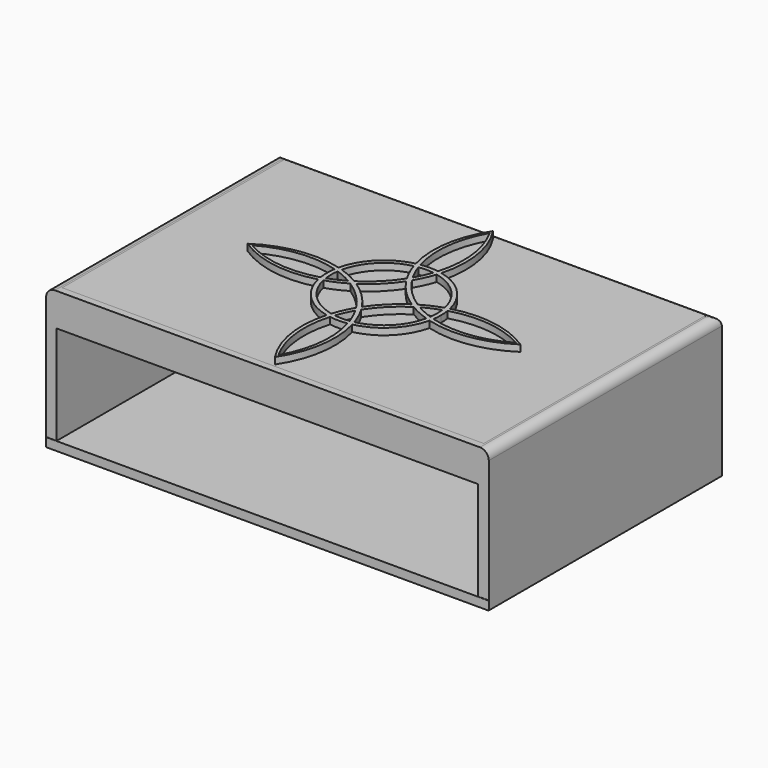
from build123d import *

# Parameters (mm, degrees)
F1_DEPTH    = 3.81
F8_DEPTH    = 81.28
F2_W        = 243.4270217588
F2_H        = 4.0062579512
F5_DEPTH    = 19.05
F2_H_2      = 160.2307879926
F6_DEPTH    = 5.08
F4_W        = 255.387352037
F4_H        = 168.597304807
F9_DEPTH    = 5.08
F7_T1_DEPTH = 193.643303895
F7_T3_DEPTH = 280.9998563766


# Not quite as in the source:
# - a fillet or chamfer that OpenCascade refuses, or shapes differently, is made with other operations: its cross-section is extruded or revolved along the edge and cut away or added


with BuildPart() as f1:
    # F0 (on Top) → F1 (new body)
    with BuildSketch(Plane.XY):
        with BuildLine():
            ThreePointArc((7.3915821042, -32.1820588837), (23.3486659148, -23.3486659148), (32.1820588837, -7.3915821042))
            ThreePointArc((32.1820588837, -7.3915821042), (30.9590231559, -7.0377991533), (29.7442225234, -6.6566978658))
            ThreePointArc((29.7442225234, -6.6566978658), (21.5526146906, -21.5526146906), (6.6566978658, -29.7442225234))
            ThreePointArc((6.6566978658, -29.7442225234), (7.0377991533, -30.9590231559), (7.3915821042, -32.1820588837))
        make_face()
        with BuildLine():
            ThreePointArc((29.7442225234, -6.6566978658), (30.9590231559, -7.0377991533), (32.1820588837, -7.3915821042))
            ThreePointArc((32.1820588837, -7.3915821042), (32.4249296069, -6.2405400398), (32.6266451411, -5.0815771994))
            ThreePointArc((32.6266451411, -5.0815771994), (31.3967387773, -4.7023200855), (30.1759000362, -4.294817459))
            ThreePointArc((30.1759000362, -4.294817459), (29.9833268944, -5.4800098856), (29.7442225234, -6.6566978658))
        make_face()
        with BuildLine():
            ThreePointArc((33.02, 0), (32.9215144135, 2.5483894364), (32.6266451411, 5.0815771994))
            ThreePointArc((32.6266451411, 5.0815771994), (31.3967387773, 4.7023200855), (30.1759000362, 4.294817459))
            ThreePointArc((30.1759000362, 4.294817459), (30.4038799588, 2.1527850447), (30.48, 0))
            ThreePointArc((30.48, 0), (30.4038799588, -2.1527850447), (30.1759000362, -4.294817459))
            ThreePointArc((30.1759000362, -4.294817459), (31.3967387773, -4.7023200855), (32.6266451411, -5.0815771994))
            ThreePointArc((32.6266451411, -5.0815771994), (32.9215144135, -2.5483894364), (33.02, 0))
        make_face()
        with BuildLine():
            ThreePointArc((78.74, 0), (56.263882639, 8.7527857998), (32.1820588837, 7.3915821042))
            ThreePointArc((32.1820588837, 7.3915821042), (32.4249296069, 6.2405400398), (32.6266451411, 5.0815771994))
            ThreePointArc((32.6266451411, 5.0815771994), (54.9332390521, 6.9989527596), (76.2, 0))
            ThreePointArc((76.2, 0), (54.9332390521, -6.9989527596), (32.6266451411, -5.0815771994))
            ThreePointArc((32.6266451411, -5.0815771994), (32.4249296069, -6.2405400398), (32.1820588837, -7.3915821042))
            ThreePointArc((32.1820588837, -7.3915821042), (56.263882639, -8.7527857998), (78.74, 0))
        make_face()
        with BuildLine():
            ThreePointArc((30.1759000362, -4.294817459), (25.3529421779, -2.367297562), (20.7299390728, 0))
            ThreePointArc((20.7299390728, 0), (19.5100699332, -0.7187762227), (18.3088168551, -1.4682500504))
            ThreePointArc((18.3088168551, -1.4682500504), (23.882724784, -4.3793997775), (29.7442225234, -6.6566978658))
            ThreePointArc((29.7442225234, -6.6566978658), (29.9833268944, -5.4800098856), (30.1759000362, -4.294817459))
        make_face()
        with BuildLine():
            ThreePointArc((30.1759000362, 4.294817459), (29.9833268944, 5.4800098856), (29.7442225234, 6.6566978658))
            ThreePointArc((29.7442225234, 6.6566978658), (23.882724784, 4.3793997775), (18.3088168551, 1.4682500504))
            ThreePointArc((18.3088168551, 1.4682500504), (19.5100699332, 0.7187762227), (20.7299390728, 0))
            ThreePointArc((20.7299390728, 0), (25.3529421779, 2.367297562), (30.1759000362, 4.294817459))
        make_face()
        with BuildLine():
            ThreePointArc((32.1820588837, 7.3915821042), (23.3486659148, 23.3486659148), (7.3915821042, 32.1820588837))
            ThreePointArc((7.3915821042, 32.1820588837), (7.0377991533, 30.9590231559), (6.6566978658, 29.7442225234))
            ThreePointArc((6.6566978658, 29.7442225234), (21.5526146906, 21.5526146906), (29.7442225234, 6.6566978658))
            ThreePointArc((29.7442225234, 6.6566978658), (30.9590231559, 7.0377991533), (32.1820588837, 7.3915821042))
        make_face()
        with BuildLine():
            ThreePointArc((32.6266451411, 5.0815771994), (32.4249296069, 6.2405400398), (32.1820588837, 7.3915821042))
            ThreePointArc((32.1820588837, 7.3915821042), (30.9590231559, 7.0377991533), (29.7442225234, 6.6566978658))
            ThreePointArc((29.7442225234, 6.6566978658), (29.9833268944, 5.4800098856), (30.1759000362, 4.294817459))
            ThreePointArc((30.1759000362, 4.294817459), (31.3967387773, 4.7023200855), (32.6266451411, 5.0815771994))
        make_face()
        with BuildLine():
            ThreePointArc((4.294817459, -30.1759000362), (5.4800098856, -29.9833268944), (6.6566978658, -29.7442225234))
            ThreePointArc((6.6566978658, -29.7442225234), (4.3793997775, -23.882724784), (1.4682500504, -18.3088168551))
            ThreePointArc((1.4682500504, -18.3088168551), (0.7187762227, -19.5100699332), (0, -20.7299390728))
            ThreePointArc((0, -20.7299390728), (2.367297562, -25.3529421779), (4.294817459, -30.1759000362))
        make_face()
        with BuildLine():
            ThreePointArc((-5.0815771994, -32.6266451411), (-6.2405400398, -32.4249296069), (-7.3915821042, -32.1820588837))
            ThreePointArc((-7.3915821042, -32.1820588837), (-8.7527857998, -56.263882639), (0, -78.74))
            ThreePointArc((0, -78.74), (8.7527857998, -56.263882639), (7.3915821042, -32.1820588837))
            ThreePointArc((7.3915821042, -32.1820588837), (6.2405400398, -32.4249296069), (5.0815771994, -32.6266451411))
            ThreePointArc((5.0815771994, -32.6266451411), (6.9989527596, -54.9332390521), (0, -76.2))
            ThreePointArc((0, -76.2), (-6.9989527596, -54.9332390521), (-5.0815771994, -32.6266451411))
        make_face()
        with BuildLine():
            ThreePointArc((-4.294817459, -30.1759000362), (-4.7023200855, -31.3967387773), (-5.0815771994, -32.6266451411))
            ThreePointArc((-5.0815771994, -32.6266451411), (0, -33.02), (5.0815771994, -32.6266451411))
            ThreePointArc((5.0815771994, -32.6266451411), (4.7023200855, -31.3967387773), (4.294817459, -30.1759000362))
            ThreePointArc((4.294817459, -30.1759000362), (0, -30.48), (-4.294817459, -30.1759000362))
        make_face()
        with BuildLine():
            ThreePointArc((5.0815771994, -32.6266451411), (6.2405400398, -32.4249296069), (7.3915821042, -32.1820588837))
            ThreePointArc((7.3915821042, -32.1820588837), (7.0377991533, -30.9590231559), (6.6566978658, -29.7442225234))
            ThreePointArc((6.6566978658, -29.7442225234), (5.4800098856, -29.9833268944), (4.294817459, -30.1759000362))
            ThreePointArc((4.294817459, -30.1759000362), (4.7023200855, -31.3967387773), (5.0815771994, -32.6266451411))
        make_face()
        with BuildLine():
            ThreePointArc((-6.6566978658, -29.7442225234), (-7.0377991533, -30.9590231559), (-7.3915821042, -32.1820588837))
            ThreePointArc((-7.3915821042, -32.1820588837), (-6.2405400398, -32.4249296069), (-5.0815771994, -32.6266451411))
            ThreePointArc((-5.0815771994, -32.6266451411), (-4.7023200855, -31.3967387773), (-4.294817459, -30.1759000362))
            ThreePointArc((-4.294817459, -30.1759000362), (-5.4800098856, -29.9833268944), (-6.6566978658, -29.7442225234))
        make_face()
        with BuildLine():
            ThreePointArc((-1.4682500504, -18.3088168551), (-4.3793997775, -23.882724784), (-6.6566978658, -29.7442225234))
            ThreePointArc((-6.6566978658, -29.7442225234), (-5.4800098856, -29.9833268944), (-4.294817459, -30.1759000362))
            ThreePointArc((-4.294817459, -30.1759000362), (-2.367297562, -25.3529421779), (0, -20.7299390728))
            ThreePointArc((0, -20.7299390728), (-0.7187762227, -19.5100699332), (-1.4682500504, -18.3088168551))
        make_face()
        with BuildLine():
            ThreePointArc((18.3088168551, -1.4682500504), (17.1314911064, -0.7483168971), (15.9719991981, 0))
            ThreePointArc((15.9719991981, 0), (7.1842048969, -7.1842048969), (0, -15.9719991981))
            ThreePointArc((0, -15.9719991981), (0.7483168971, -17.1314911064), (1.4682500504, -18.3088168551))
            ThreePointArc((1.4682500504, -18.3088168551), (8.9802561211, -8.9802561211), (18.3088168551, -1.4682500504))
        make_face()
        with BuildLine():
            ThreePointArc((18.3088168551, 1.4682500504), (8.9802561211, 8.9802561211), (1.4682500504, 18.3088168551))
            ThreePointArc((1.4682500504, 18.3088168551), (0.7483168971, 17.1314911064), (0, 15.9719991981))
            ThreePointArc((0, 15.9719991981), (7.1842048969, 7.1842048969), (15.9719991981, 0))
            ThreePointArc((15.9719991981, 0), (17.1314911064, 0.7483168971), (18.3088168551, 1.4682500504))
        make_face()
        with BuildLine():
            ThreePointArc((0, 15.9719991981), (-0.7483168971, 17.1314911064), (-1.4682500504, 18.3088168551))
            ThreePointArc((-1.4682500504, 18.3088168551), (-8.9802561211, 8.9802561211), (-18.3088168551, 1.4682500504))
            ThreePointArc((-18.3088168551, 1.4682500504), (-17.1314911064, 0.7483168971), (-15.9719991981, 0))
            ThreePointArc((-15.9719991981, 0), (-7.1842048969, 7.1842048969), (0, 15.9719991981))
        make_face()
        with BuildLine():
            ThreePointArc((0, -15.9719991981), (-7.1842048969, -7.1842048969), (-15.9719991981, 0))
            ThreePointArc((-15.9719991981, 0), (-17.1314911064, -0.7483168971), (-18.3088168551, -1.4682500504))
            ThreePointArc((-18.3088168551, -1.4682500504), (-8.9802561211, -8.9802561211), (-1.4682500504, -18.3088168551))
            ThreePointArc((-1.4682500504, -18.3088168551), (-0.7483168971, -17.1314911064), (0, -15.9719991981))
        make_face()
        with BuildLine():
            ThreePointArc((-18.3088168551, 1.4682500504), (-23.882724784, 4.3793997775), (-29.7442225234, 6.6566978658))
            ThreePointArc((-29.7442225234, 6.6566978658), (-29.9833268944, 5.4800098856), (-30.1759000362, 4.294817459))
            ThreePointArc((-30.1759000362, 4.294817459), (-25.3529421779, 2.367297562), (-20.7299390728, 0))
            ThreePointArc((-20.7299390728, 0), (-19.5100699332, 0.7187762227), (-18.3088168551, 1.4682500504))
        make_face()
        with BuildLine():
            ThreePointArc((-18.3088168551, -1.4682500504), (-19.5100699332, -0.7187762227), (-20.7299390728, 0))
            ThreePointArc((-20.7299390728, 0), (-25.3529421779, -2.367297562), (-30.1759000362, -4.294817459))
            ThreePointArc((-30.1759000362, -4.294817459), (-29.9833268944, -5.4800098856), (-29.7442225234, -6.6566978658))
            ThreePointArc((-29.7442225234, -6.6566978658), (-23.882724784, -4.3793997775), (-18.3088168551, -1.4682500504))
        make_face()
        with BuildLine():
            ThreePointArc((-30.1759000362, 4.294817459), (-31.3967387773, 4.7023200855), (-32.6266451411, 5.0815771994))
            ThreePointArc((-32.6266451411, 5.0815771994), (-33.02, 0), (-32.6266451411, -5.0815771994))
            ThreePointArc((-32.6266451411, -5.0815771994), (-31.3967387773, -4.7023200855), (-30.1759000362, -4.294817459))
            ThreePointArc((-30.1759000362, -4.294817459), (-30.48, 0), (-30.1759000362, 4.294817459))
        make_face()
        with BuildLine():
            ThreePointArc((-32.6266451411, -5.0815771994), (-32.4249296069, -6.2405400398), (-32.1820588837, -7.3915821042))
            ThreePointArc((-32.1820588837, -7.3915821042), (-30.9590231559, -7.0377991533), (-29.7442225234, -6.6566978658))
            ThreePointArc((-29.7442225234, -6.6566978658), (-29.9833268944, -5.4800098856), (-30.1759000362, -4.294817459))
            ThreePointArc((-30.1759000362, -4.294817459), (-31.3967387773, -4.7023200855), (-32.6266451411, -5.0815771994))
        make_face()
        with BuildLine():
            ThreePointArc((-29.7442225234, -6.6566978658), (-30.9590231559, -7.0377991533), (-32.1820588837, -7.3915821042))
            ThreePointArc((-32.1820588837, -7.3915821042), (-23.3486659148, -23.3486659148), (-7.3915821042, -32.1820588837))
            ThreePointArc((-7.3915821042, -32.1820588837), (-7.0377991533, -30.9590231559), (-6.6566978658, -29.7442225234))
            ThreePointArc((-6.6566978658, -29.7442225234), (-21.5526146906, -21.5526146906), (-29.7442225234, -6.6566978658))
        make_face()
        with BuildLine():
            ThreePointArc((-29.7442225234, 6.6566978658), (-30.9590231559, 7.0377991533), (-32.1820588837, 7.3915821042))
            ThreePointArc((-32.1820588837, 7.3915821042), (-32.4249296069, 6.2405400398), (-32.6266451411, 5.0815771994))
            ThreePointArc((-32.6266451411, 5.0815771994), (-31.3967387773, 4.7023200855), (-30.1759000362, 4.294817459))
            ThreePointArc((-30.1759000362, 4.294817459), (-29.9833268944, 5.4800098856), (-29.7442225234, 6.6566978658))
        make_face()
        with BuildLine():
            ThreePointArc((-32.6266451411, 5.0815771994), (-32.4249296069, 6.2405400398), (-32.1820588837, 7.3915821042))
            ThreePointArc((-32.1820588837, 7.3915821042), (-56.263882639, 8.7527857998), (-78.74, 0))
            ThreePointArc((-78.74, 0), (-56.263882639, -8.7527857998), (-32.1820588837, -7.3915821042))
            ThreePointArc((-32.1820588837, -7.3915821042), (-32.4249296069, -6.2405400398), (-32.6266451411, -5.0815771994))
            ThreePointArc((-32.6266451411, -5.0815771994), (-54.9332390521, -6.9989527596), (-76.2, 0))
            ThreePointArc((-76.2, 0), (-54.9332390521, 6.9989527596), (-32.6266451411, 5.0815771994))
        make_face()
        with BuildLine():
            ThreePointArc((-6.6566978658, 29.7442225234), (-7.0377991533, 30.9590231559), (-7.3915821042, 32.1820588837))
            ThreePointArc((-7.3915821042, 32.1820588837), (-23.3486659148, 23.3486659148), (-32.1820588837, 7.3915821042))
            ThreePointArc((-32.1820588837, 7.3915821042), (-30.9590231559, 7.0377991533), (-29.7442225234, 6.6566978658))
            ThreePointArc((-29.7442225234, 6.6566978658), (-21.5526146906, 21.5526146906), (-6.6566978658, 29.7442225234))
        make_face()
        with BuildLine():
            ThreePointArc((0, 20.7299390728), (-2.367297562, 25.3529421779), (-4.294817459, 30.1759000362))
            ThreePointArc((-4.294817459, 30.1759000362), (-5.4800098856, 29.9833268944), (-6.6566978658, 29.7442225234))
            ThreePointArc((-6.6566978658, 29.7442225234), (-4.3793997775, 23.882724784), (-1.4682500504, 18.3088168551))
            ThreePointArc((-1.4682500504, 18.3088168551), (-0.7187762227, 19.5100699332), (0, 20.7299390728))
        make_face()
        with BuildLine():
            ThreePointArc((6.6566978658, 29.7442225234), (5.4800098856, 29.9833268944), (4.294817459, 30.1759000362))
            ThreePointArc((4.294817459, 30.1759000362), (2.367297562, 25.3529421779), (0, 20.7299390728))
            ThreePointArc((0, 20.7299390728), (0.7187762227, 19.5100699332), (1.4682500504, 18.3088168551))
            ThreePointArc((1.4682500504, 18.3088168551), (4.3793997775, 23.882724784), (6.6566978658, 29.7442225234))
        make_face()
        with BuildLine():
            ThreePointArc((5.0815771994, 32.6266451411), (0, 33.02), (-5.0815771994, 32.6266451411))
            ThreePointArc((-5.0815771994, 32.6266451411), (-4.7023200855, 31.3967387773), (-4.294817459, 30.1759000362))
            ThreePointArc((-4.294817459, 30.1759000362), (0, 30.48), (4.294817459, 30.1759000362))
            ThreePointArc((4.294817459, 30.1759000362), (4.7023200855, 31.3967387773), (5.0815771994, 32.6266451411))
        make_face()
        with BuildLine():
            ThreePointArc((-5.0815771994, 32.6266451411), (-6.9989527596, 54.9332390521), (0, 76.2))
            ThreePointArc((0, 76.2), (6.9989527596, 54.9332390521), (5.0815771994, 32.6266451411))
            ThreePointArc((5.0815771994, 32.6266451411), (6.2405400398, 32.4249296069), (7.3915821042, 32.1820588837))
            ThreePointArc((7.3915821042, 32.1820588837), (8.7527857998, 56.263882639), (0, 78.74))
            ThreePointArc((0, 78.74), (-8.7527857998, 56.263882639), (-7.3915821042, 32.1820588837))
            ThreePointArc((-7.3915821042, 32.1820588837), (-6.2405400398, 32.4249296069), (-5.0815771994, 32.6266451411))
        make_face()
        with BuildLine():
            ThreePointArc((7.3915821042, 32.1820588837), (6.2405400398, 32.4249296069), (5.0815771994, 32.6266451411))
            ThreePointArc((5.0815771994, 32.6266451411), (4.7023200855, 31.3967387773), (4.294817459, 30.1759000362))
            ThreePointArc((4.294817459, 30.1759000362), (5.4800098856, 29.9833268944), (6.6566978658, 29.7442225234))
            ThreePointArc((6.6566978658, 29.7442225234), (7.0377991533, 30.9590231559), (7.3915821042, 32.1820588837))
        make_face()
        with BuildLine():
            ThreePointArc((1.4682500504, 18.3088168551), (0.7187762227, 19.5100699332), (0, 20.7299390728))
            ThreePointArc((0, 20.7299390728), (-0.7187762227, 19.5100699332), (-1.4682500504, 18.3088168551))
            ThreePointArc((-1.4682500504, 18.3088168551), (-0.7483168971, 17.1314911064), (0, 15.9719991981))
            ThreePointArc((0, 15.9719991981), (0.7483168971, 17.1314911064), (1.4682500504, 18.3088168551))
        make_face()
        with BuildLine():
            ThreePointArc((-4.294817459, 30.1759000362), (-4.7023200855, 31.3967387773), (-5.0815771994, 32.6266451411))
            ThreePointArc((-5.0815771994, 32.6266451411), (-6.2405400398, 32.4249296069), (-7.3915821042, 32.1820588837))
            ThreePointArc((-7.3915821042, 32.1820588837), (-7.0377991533, 30.9590231559), (-6.6566978658, 29.7442225234))
            ThreePointArc((-6.6566978658, 29.7442225234), (-5.4800098856, 29.9833268944), (-4.294817459, 30.1759000362))
        make_face()
        with BuildLine():
            ThreePointArc((-15.9719991981, 0), (-17.1314911064, 0.7483168971), (-18.3088168551, 1.4682500504))
            ThreePointArc((-18.3088168551, 1.4682500504), (-19.5100699332, 0.7187762227), (-20.7299390728, 0))
            ThreePointArc((-20.7299390728, 0), (-19.5100699332, -0.7187762227), (-18.3088168551, -1.4682500504))
            ThreePointArc((-18.3088168551, -1.4682500504), (-17.1314911064, -0.7483168971), (-15.9719991981, 0))
        make_face()
        with BuildLine():
            ThreePointArc((1.4682500504, -18.3088168551), (0.7483168971, -17.1314911064), (0, -15.9719991981))
            ThreePointArc((0, -15.9719991981), (-0.7483168971, -17.1314911064), (-1.4682500504, -18.3088168551))
            ThreePointArc((-1.4682500504, -18.3088168551), (-0.7187762227, -19.5100699332), (0, -20.7299390728))
            ThreePointArc((0, -20.7299390728), (0.7187762227, -19.5100699332), (1.4682500504, -18.3088168551))
        make_face()
        with BuildLine():
            ThreePointArc((20.7299390728, 0), (19.5100699332, 0.7187762227), (18.3088168551, 1.4682500504))
            ThreePointArc((18.3088168551, 1.4682500504), (17.1314911064, 0.7483168971), (15.9719991981, 0))
            ThreePointArc((15.9719991981, 0), (17.1314911064, -0.7483168971), (18.3088168551, -1.4682500504))
            ThreePointArc((18.3088168551, -1.4682500504), (19.5100699332, -0.7187762227), (20.7299390728, 0))
        make_face()
    extrude(amount=F1_DEPTH)


with BuildPart() as f8:
    # F2 (on Top) → F8 (new body)
    with BuildSketch(Plane.XY):
        Polygon((127.7999281883, -84.1216519475), (127.7999281883, 84.1216519475), (-127.7999281883, 84.1216519475), (-127.7999281883, -84.1216519475), (-121.7135108794, -84.1216519475), (-121.7135108794, -80.1153939963), (-121.7135108794, 80.1153939963), (121.7135108794, 80.1153939963), (121.7135108794, -80.1153939963), (121.7135108794, -84.1216519475), align=None)
    extrude(amount=-F8_DEPTH)

    # F2 (on Top) → F5 (join)
    with BuildSketch(Plane.XY):
        with Locations((0, -82.1185229719)):
            Rectangle(F2_W, F2_H)
    extrude(amount=-F5_DEPTH)

    # F4 (on offset) → F9 (join)
    with BuildSketch(Plane.XY.offset(-76.2)):
        Rectangle(F4_W, F4_H)
    extrude(amount=-F9_DEPTH)

    # F7: fillet of radius 5.08 on 3 edges, made by hand

    # F7_s2 → F7_t1 (cut)
    with BuildSketch(Plane.XZ.offset(-96.8216519475)):
        with BuildLine():
            ThreePointArc((127.7999281883, -5.08), (126.3120306368, -1.4878975516), (122.7199281883, 0))
            Line((122.7199281883, 0), (127.7999281883, 0))
            Line((127.7999281883, 0), (127.7999281883, -5.08))
        make_face()
        with BuildLine():
            ThreePointArc((-122.7199281883, 0), (-126.3120306368, -1.4878975516), (-127.7999281883, -5.08))
            Line((-127.7999281883, -5.08), (-127.7999281883, 0))
            Line((-127.7999281883, 0), (-122.7199281883, 0))
        make_face()
    extrude(amount=F7_T1_DEPTH, mode=Mode.SUBTRACT)

    # F7_s4 → F7_t3 (cut)
    with BuildSketch(Plane.YZ.offset(-140.4999281883)):
        with BuildLine():
            ThreePointArc((84.1216519475, -5.08), (82.6337543959, -1.4878975516), (79.0416519475, 0))
            Line((79.0416519475, 0), (84.1216519475, 0))
            Line((84.1216519475, 0), (84.1216519475, -5.08))
        make_face()
    extrude(amount=F7_T3_DEPTH, mode=Mode.SUBTRACT)


with BuildPart() as f6:
    # F2 (on Top) → F6 (new body)
    with BuildSketch(Plane.XY):
        Rectangle(F2_W, F2_H_2)
    extrude(amount=-F6_DEPTH)


solid = Compound([f1.part, f8.part, f6.part])
